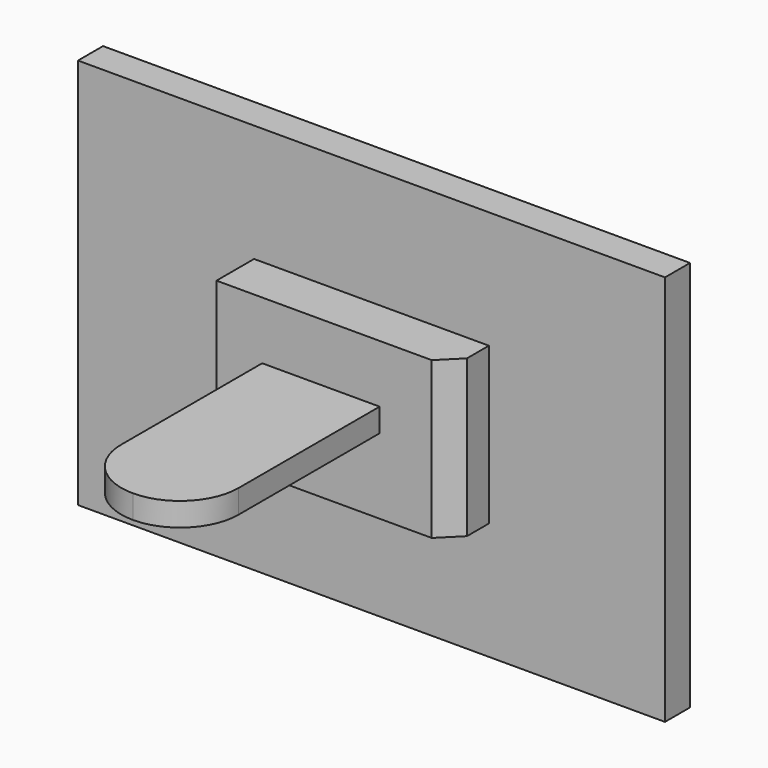
from build123d import *

# Parameters (mm, degrees)
F0_W     = 150
F0_H     = 100
F1_DEPTH = 3
F2_DEPTH = 5
F3_W     = 60
F3_H     = 40
F4_DEPTH = 10
F5_DEPTH = 10
F6_SIZE  = 5
F7_W     = 30
F7_H     = 60
F8_DEPTH = 6
F9_R     = 14.99999


# Not quite as in the source:
# - a fillet or chamfer is up to 0.001 mm smaller than in the source, because OpenCascade refuses the exact size


with BuildPart() as f1:
    # F0 (on Front) → F1 (new body)
    with BuildSketch(Plane.XZ):
        Rectangle(F0_W, F0_H)
    extrude(amount=F1_DEPTH)

    # F2 (add): a face of the model
    f2_faces = [f1.faces().sort_by_distance(p)[0] for p in [
        (0, -3, 0),
    ]]
    extrude(f2_faces, amount=F2_DEPTH)

    # F3 (on Front) → F4 (join)
    with BuildSketch(Plane.XZ):
        Rectangle(F3_W, F3_H)
    extrude(amount=F4_DEPTH)

    # F5 (add): a face of the model
    f5_faces = [f1.faces().sort_by_distance(p)[0] for p in [
        (0, -10, 0),
    ]]
    extrude(f5_faces, amount=F5_DEPTH)

    # F6
    f6_edges = [f1.edges().sort_by_distance(p)[0] for p in [
        (30, -20, 0),
    ]]
    chamfer(f6_edges, length=F6_SIZE)


with BuildPart() as f8:
    # F7 (on Top) → F8 (new body)
    with BuildSketch(Plane.XY):
        with Locations((-2.3789281398, -51.1790004373)):
            Rectangle(F7_W, F7_H)
    extrude(amount=F8_DEPTH)

    # F9 (radius 15 in the source; OpenCascade refuses exactly that, so slightly less here)
    f9_edges = [f8.edges().sort_by_distance(p)[0] for p in [
        (12.621072, -81.179, 3),
        (-17.378928, -81.179, 3),
    ]]
    fillet(f9_edges, radius=F9_R)


solid = Compound([f1.part, f8.part])
